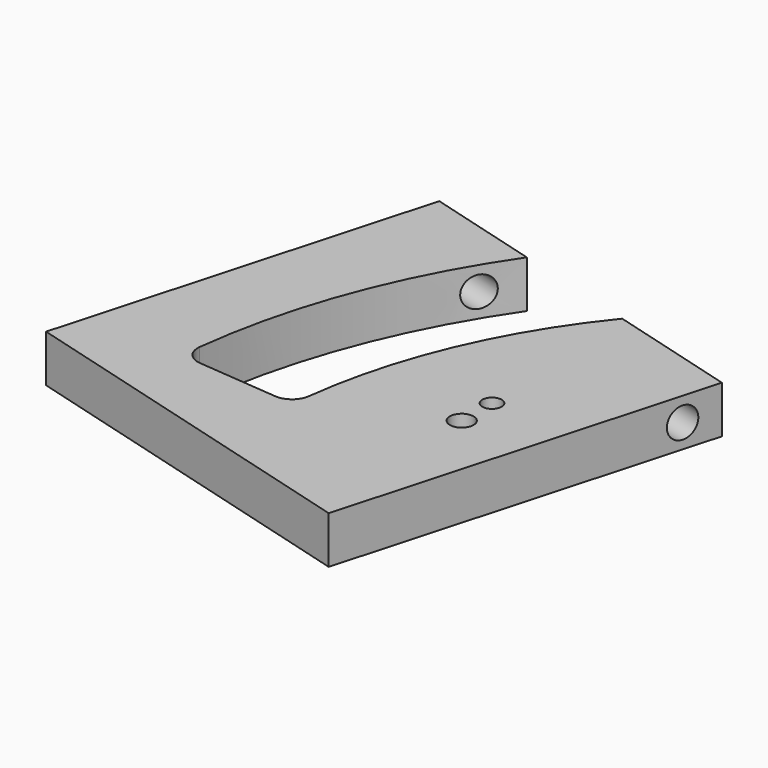
from build123d import *

# Parameters (mm, degrees)
F0_R     = 6.25
F0_R_2   = 5.1
F1_DEPTH = 25
F2_R     = 10
F3_R     = 8
F4_DEPTH = 200


# Not quite as in the source:
# - a feature names something its author has since deleted; it is built from what else it names


with BuildPart() as f1:
    # F0 (on Top) → F1 (new body)
    with BuildSketch(Plane.XY):
        with BuildLine():
            ThreePointArc((-1.8786394122, 86.9422913227), (-42.1479963116, 19.0841411618), (-60.6516929848, -57.622852377))
            Line((-60.6516929848, -57.622852377), (-123.4119589646, -52.1320405839))
            ThreePointArc((-123.4119589646, -52.1320405839), (-105.3496683323, 30.162565727), (-66.9193045914, 105.1409340308))
            Line((-66.9193045914, 105.1409340308), (-126.574214908, 121.8326206187))
            Line((-126.574214908, 121.8326206187), (-180.4652056167, -70.7699783265))
            Line((-180.4652056167, -70.7699783265), (12.1373933285, -124.6609690352))
            Line((12.1373933285, -124.6609690352), (66.0283840372, 67.9416299099))
            Line((66.0283840372, 67.9416299099), (-1.8786394122, 86.9422913227))
        make_face()
        with Locations((3.3399020095, -25.7191242051)):
            Circle(F0_R, mode=Mode.SUBTRACT)
        with Locations((3.3399020095, -5.7191242051)):
            Circle(F0_R_2, mode=Mode.SUBTRACT)
    extrude(amount=F1_DEPTH)

    # F2
    f2_edges = [f1.edges().sort_by_distance(p)[0] for p in [
        (-123.411959, -52.132041, 12.5),
        (-60.651693, -57.622852, 12.5),
    ]]
    fillet(f2_edges, radius=F2_R)

    # F3 (on face) → F4 (cut, through all)
    with BuildSketch(Plane(origin=(-148.998349815, 41.6903444163, 0), x_dir=(-0.2694549535, -0.9630129947, 0), z_dir=(-0.9630129947, 0.2694549535, 0))):
        with Locations((-63.2203476394, 12.5)):
            Circle(F3_R)
    extrude(amount=-F4_DEPTH, mode=Mode.SUBTRACT)


solid = f1.part
